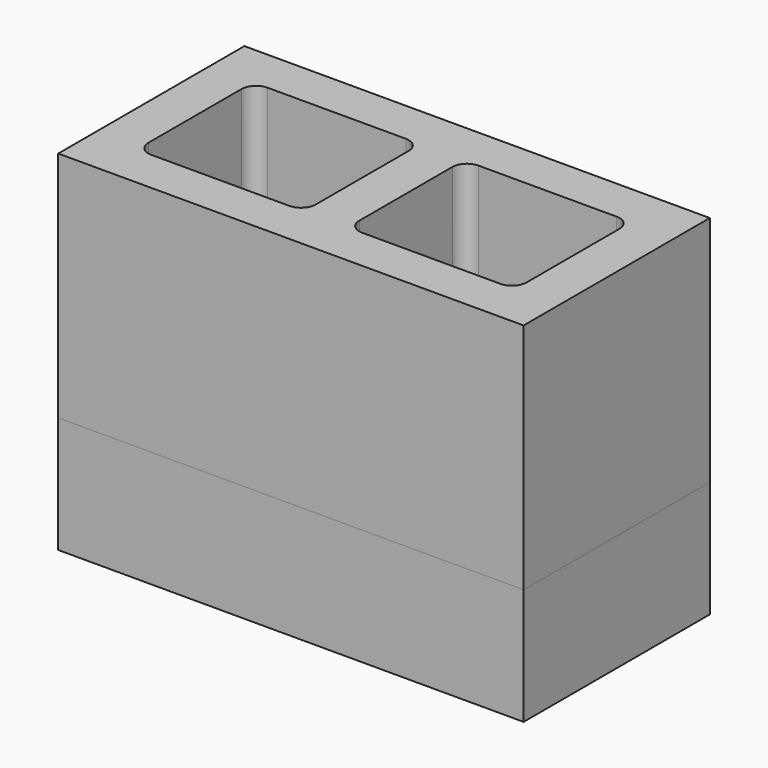
from build123d import *

# Parameters (mm, degrees)
F1_W     = 406.4
F1_H     = 203.2
F2_DEPTH = 203.2
F3_DEPTH = 101.6


# Not quite as in the source:
# - a variable given as a bare number and used for a length is read in inches; the dataset says mm whatever the document's units were


with BuildPart() as f2:
    # F1 (on Top) → F2 (new body)
    with BuildSketch(Plane.XY):
        Rectangle(F1_W, F1_H)
        with BuildLine():
            ThreePointArc((-165.1, 50.8), (-161.3802561211, 59.7802561211), (-152.4, 63.5))
            Line((-152.4, 63.5), (-31.75, 63.5))
            ThreePointArc((-31.75, 63.5), (-22.7697438789, 59.7802561211), (-19.05, 50.8))
            Line((-19.05, 50.8), (-19.05, -50.8))
            ThreePointArc((-19.05, -50.8), (-22.7697438789, -59.7802561211), (-31.75, -63.5))
            Line((-31.75, -63.5), (-152.4, -63.5))
            ThreePointArc((-152.4, -63.5), (-161.3802561211, -59.7802561211), (-165.1, -50.8))
            Line((-165.1, -50.8), (-165.1, 50.8))
        make_face(mode=Mode.SUBTRACT)
        with BuildLine():
            Line((19.05, -50.8), (19.05, 50.8))
            ThreePointArc((19.05, 50.8), (22.7697438789, 59.7802561211), (31.75, 63.5))
            Line((31.75, 63.5), (152.4, 63.5))
            ThreePointArc((152.4, 63.5), (161.3802561211, 59.7802561211), (165.1, 50.8))
            Line((165.1, 50.8), (165.1, -50.8))
            ThreePointArc((165.1, -50.8), (161.3802561211, -59.7802561211), (152.4, -63.5))
            Line((152.4, -63.5), (31.75, -63.5))
            ThreePointArc((31.75, -63.5), (22.7697438789, -59.7802561211), (19.05, -50.8))
        make_face(mode=Mode.SUBTRACT)
    extrude(amount=F2_DEPTH)


with BuildPart() as f3:
    # F1 (on Top) → F3 (new body)
    with BuildSketch(Plane.XY):
        Rectangle(F1_W, F1_H)
        with BuildLine():
            ThreePointArc((-165.1, 50.8), (-161.3802561211, 59.7802561211), (-152.4, 63.5))
            Line((-152.4, 63.5), (-31.75, 63.5))
            ThreePointArc((-31.75, 63.5), (-22.7697438789, 59.7802561211), (-19.05, 50.8))
            Line((-19.05, 50.8), (-19.05, -50.8))
            ThreePointArc((-19.05, -50.8), (-22.7697438789, -59.7802561211), (-31.75, -63.5))
            Line((-31.75, -63.5), (-152.4, -63.5))
            ThreePointArc((-152.4, -63.5), (-161.3802561211, -59.7802561211), (-165.1, -50.8))
            Line((-165.1, -50.8), (-165.1, 50.8))
        make_face(mode=Mode.SUBTRACT)
        with BuildLine():
            Line((19.05, -50.8), (19.05, 50.8))
            ThreePointArc((19.05, 50.8), (22.7697438789, 59.7802561211), (31.75, 63.5))
            Line((31.75, 63.5), (152.4, 63.5))
            ThreePointArc((152.4, 63.5), (161.3802561211, 59.7802561211), (165.1, 50.8))
            Line((165.1, 50.8), (165.1, -50.8))
            ThreePointArc((165.1, -50.8), (161.3802561211, -59.7802561211), (152.4, -63.5))
            Line((152.4, -63.5), (31.75, -63.5))
            ThreePointArc((31.75, -63.5), (22.7697438789, -59.7802561211), (19.05, -50.8))
        make_face(mode=Mode.SUBTRACT)
        with BuildLine():
            Line((-31.75, 63.5), (-152.4, 63.5))
            ThreePointArc((-152.4, 63.5), (-161.3802561211, 59.7802561211), (-165.1, 50.8))
            Line((-165.1, 50.8), (-165.1, -50.8))
            ThreePointArc((-165.1, -50.8), (-161.3802561211, -59.7802561211), (-152.4, -63.5))
            Line((-152.4, -63.5), (-31.75, -63.5))
            ThreePointArc((-31.75, -63.5), (-22.7697438789, -59.7802561211), (-19.05, -50.8))
            Line((-19.05, -50.8), (-19.05, 50.8))
            ThreePointArc((-19.05, 50.8), (-22.7697438789, 59.7802561211), (-31.75, 63.5))
        make_face()
        with BuildLine():
            ThreePointArc((31.75, 63.5), (22.7697438789, 59.7802561211), (19.05, 50.8))
            Line((19.05, 50.8), (19.05, -50.8))
            ThreePointArc((19.05, -50.8), (22.7697438789, -59.7802561211), (31.75, -63.5))
            Line((31.75, -63.5), (152.4, -63.5))
            ThreePointArc((152.4, -63.5), (161.3802561211, -59.7802561211), (165.1, -50.8))
            Line((165.1, -50.8), (165.1, 50.8))
            ThreePointArc((165.1, 50.8), (161.3802561211, 59.7802561211), (152.4, 63.5))
            Line((152.4, 63.5), (31.75, 63.5))
        make_face()
    extrude(amount=-F3_DEPTH)


solid = Compound([f2.part, f3.part])
